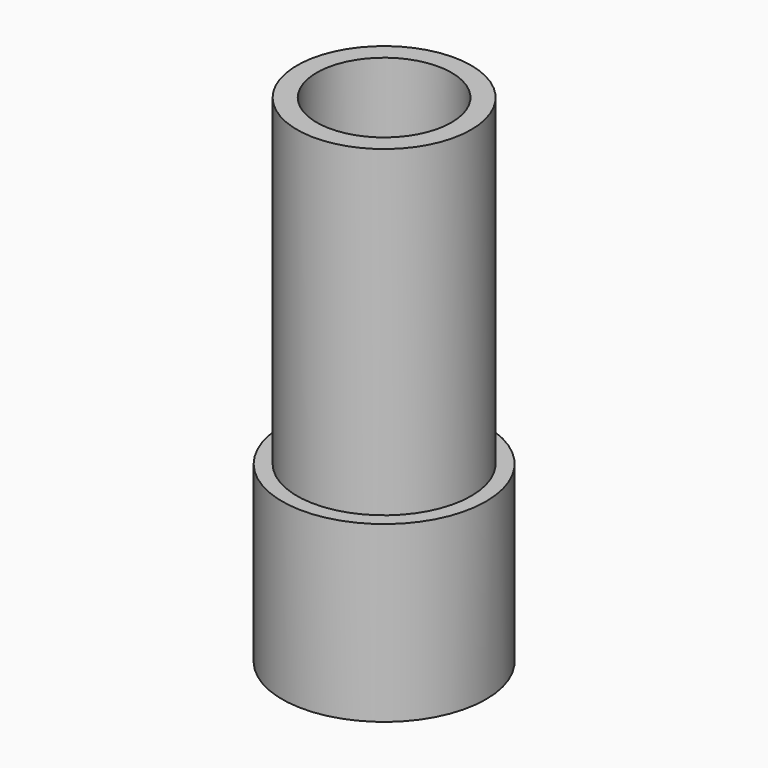
from build123d import *

# Parameters (mm, degrees)
F0_R      = 34.925
F0_R_2    = 29.845
F1_DEPTH  = 59.69
F7_R      = 29.845
F7_R_2    = 24.8583947088
F8_DEPTH  = 69.85
F15_R     = 29.845
F15_R_2   = 23.114
F16_DEPTH = 54.61


# Not quite as in the source:
# - the program builds the solid bodies; features that only make, move or delete a surface that nothing else refers to are left out


with BuildPart() as f1:
    # F0 (on Top) → F1 (new body)
    with BuildSketch(Plane.XY):
        Circle(F0_R)
        Circle(F0_R_2, mode=Mode.SUBTRACT)
    extrude(amount=F1_DEPTH)

    # F7 (on offset) → F8 (join)
    with BuildSketch(Plane.XY.offset(45.72)):
        Circle(F7_R)
        Circle(F7_R_2, mode=Mode.SUBTRACT)
    extrude(amount=F8_DEPTH)

    # F15 (on offset) → F16 (join)
    with BuildSketch(Plane.XY.offset(115.57)):
        Circle(F15_R)
        Circle(F15_R_2, mode=Mode.SUBTRACT)
    extrude(amount=F16_DEPTH)


solid = f1.part
